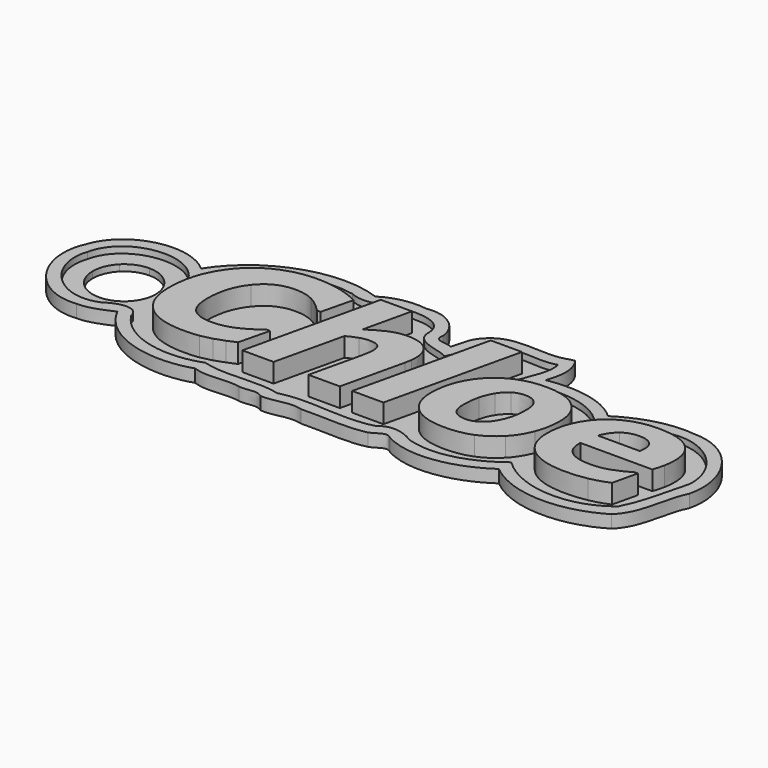
from build123d import *

# Parameters (mm, degrees)
F1_DEPTH = 4
F2_DEPTH = 1
F3_DEPTH = 2
F4_DEPTH = 1


# Not quite as in the source:
# - ends of sketch curves that miss each other by under 0.0002 mm in the source are joined


with BuildPart() as f1:
    # F0 (on Top) → F1 (new body)
    with BuildSketch(Plane.XY):
        with BuildLine():
            add(Edge.make_bspline(
                [(-23.2617298845, -10.9770997937), (-25.988726302, -10.9770997937), (-28.092665777, -10.3088950788), (-29.5735483095, -8.972486227)],
                knots=[0, 0, 0, 0, 1, 1, 1, 1], degree=3))
            add(Edge.make_bspline(
                [(-20.9049541001, -10.8281063081), (-21.4648019653, -10.9274351059), (-22.2503938934, -10.9770997937), (-23.2617298845, -10.9770997937)],
                knots=[0, 0, 0, 0, 1, 1, 1, 1], degree=3))
            add(Edge.make_bspline(
                [(-19.0764216423, -10.3946765976), (-19.7265679417, -10.5843038297), (-20.336078761, -10.7287803998), (-20.9049541001, -10.8281063081)],
                knots=[0, 0, 0, 0, 1, 1, 1, 1], degree=3))
            add(Edge.make_bspline(
                [(-17.5187839092, -9.8393456479), (-18.0605733589, -10.0650897109), (-18.579785744, -10.2502000274), (-19.0764216423, -10.3946765976)],
                knots=[0, 0, 0, 0, 1, 1, 1, 1], degree=3))
            add(Edge.make_bspline(
                [(-16.0965935386, -9.2433809518), (-16.5029338922, -9.4059159375), (-16.976997349, -9.6045706435), (-17.5187839092, -9.8393456479)],
                knots=[0, 0, 0, 0, 1, 1, 1, 1], degree=3))
            Line((-16.0965935386, -9.2433809518), (-14.9182056464, -4.4214742671))
            Line((-14.9182056464, -4.4214742671), (-15.4599950961, -4.4214742671))
            add(Edge.make_bspline(
                [(-18.561724439, -6.344820341), (-17.4691209551, -5.8391506117), (-16.4352113668, -5.1980352538), (-15.4599950961, -4.4214742671)],
                knots=[0, 0, 0, 0, 1, 1, 1, 1], degree=3))
            add(Edge.make_bspline(
                [(-22.0697958691, -7.0897785227), (-20.8236883411, -7.0897785227), (-19.6543308124, -6.8414591288), (-18.561724439, -6.344820341)],
                knots=[0, 0, 0, 0, 1, 1, 1, 1], degree=3))
            add(Edge.make_bspline(
                [(-25.2392512048, -6.0062042466), (-24.516868354, -6.7285870973), (-23.4603834348, -7.0897785227), (-22.0697958691, -7.0897785227)],
                knots=[0, 0, 0, 0, 1, 1, 1, 1], degree=3))
            add(Edge.make_bspline(
                [(-26.322825481, -2.5116743164), (-26.322825481, -4.1189778931), (-25.9616340556, -5.2838213958), (-25.2392512048, -6.0062042466)],
                knots=[0, 0, 0, 0, 1, 1, 1, 1], degree=3))
            add(Edge.make_bspline(
                [(-24.3723917839, 3.6646967461), (-25.6726809153, 2.0483651175), (-26.322825481, -0.0104248514), (-26.322825481, -2.5116743164)],
                knots=[0, 0, 0, 0, 1, 1, 1, 1], degree=3))
            add(Edge.make_bspline(
                [(-19.3879501135, 6.0891939001), (-21.4015946217, 6.0891939001), (-23.0630751785, 5.2810283747), (-24.3723917839, 3.6646967461)],
                knots=[0, 0, 0, 0, 1, 1, 1, 1], degree=3))
            add(Edge.make_bspline(
                [(-16.3945758866, 5.4390493344), (-17.2433768921, 5.8724790449), (-18.2411684937, 6.0891939001), (-19.3879501135, 6.0891939001)],
                knots=[0, 0, 0, 0, 1, 1, 1, 1], degree=3))
            add(Edge.make_bspline(
                [(-13.8346313703, 3.4073481445), (-14.6924633172, 4.3283857013), (-15.5457777707, 5.0056196239), (-16.3945758866, 5.4390493344)],
                knots=[0, 0, 0, 0, 1, 1, 1, 1], degree=3))
            Line((-13.8346313703, 3.4073481445), (-13.2386666742, 3.4073481445))
            Line((-13.2386666742, 3.4073481445), (-12.046737282, 8.2969761988))
            add(Edge.make_bspline(
                [(-15.2703678641, 9.5430900839), (-14.0784384719, 9.2631644176), (-13.0038951372, 8.8477931225), (-12.046737282, 8.2969761988)],
                knots=[0, 0, 0, 0, 1, 1, 1, 1], degree=3))
            add(Edge.make_bspline(
                [(-19.1441476351, 9.9765197943), (-17.7535600694, 9.9765197943), (-16.4623001458, 9.8320432242), (-15.2703678641, 9.5430900839)],
                knots=[0, 0, 0, 0, 1, 1, 1, 1], degree=3))
            add(Edge.make_bspline(
                [(-24.0879555591, 9.0148467574), (-22.5167717028, 9.6559621153), (-20.8688355355, 9.9765197943), (-19.1441476351, 9.9765197943)],
                knots=[0, 0, 0, 0, 1, 1, 1, 1], degree=3))
            add(Edge.make_bspline(
                [(-28.1107241925, 6.3465425017), (-26.9910313517, 7.4842966475), (-25.6501084739, 8.3737313994), (-24.0879555591, 9.0148467574)],
                knots=[0, 0, 0, 0, 1, 1, 1, 1], degree=3))
            add(Edge.make_bspline(
                [(-30.8196621945, 2.1747850059), (-30.1604855315, 3.7820856931), (-29.2575058123, 5.172671525), (-28.1107241925, 6.3465425017)],
                knots=[0, 0, 0, 0, 1, 1, 1, 1], degree=3))
            add(Edge.make_bspline(
                [(-31.7948767314, -3.2024526285), (-31.7948767314, -1.2249313082), (-31.4698050265, 0.5674814292), (-30.8196621945, 2.1747850059)],
                knots=[0, 0, 0, 0, 1, 1, 1, 1], degree=3))
            add(Edge.make_bspline(
                [(-29.5735483095, -8.972486227), (-31.0544337315, -7.6270493232), (-31.7948767314, -5.703704983), (-31.7948767314, -3.2024526285)],
                knots=[0, 0, 0, 0, 1, 1, 1, 1], degree=3))
        make_face()
    extrude(amount=F1_DEPTH)



with BuildPart() as f1b:
    # F0 (on Top) → F1, piece 2 (new body)
    with BuildSketch(Plane.XY):
        with BuildLine():
            add(Edge.make_bspline(
                [(3.4740269711, 1.1860197225), (3.4740269711, 0.969306601), (3.455966822, 0.6893838242), (3.4198471015, 0.346252548)],
                knots=[0, 0, 0, 0, 1, 1, 1, 1], degree=3))
            add(Edge.make_bspline(
                [(2.3498189486, 4.030405087), (3.0992911563, 3.3622003721), (3.4740269711, 2.4140723026), (3.4740269711, 1.1860197225)],
                knots=[0, 0, 0, 0, 1, 1, 1, 1], degree=3))
            add(Edge.make_bspline(
                [(-0.8467286336, 5.0462533703), (0.5348279907, 5.0462533703), (1.6003438514, 4.7076372759), (2.3498189486, 4.030405087)],
                knots=[0, 0, 0, 0, 1, 1, 1, 1], degree=3))
            add(Edge.make_bspline(
                [(-3.5827542588, 4.4909224207), (-2.7520116688, 4.8611430538), (-1.8400033197, 5.0462533703), (-0.8467286336, 5.0462533703)],
                knots=[0, 0, 0, 0, 1, 1, 1, 1], degree=3))
            add(Edge.make_bspline(
                [(-6.3187752608, 2.9468308108), (-5.3255005747, 3.6060045843), (-4.4134939593, 4.1207017875), (-3.5827542588, 4.4909224207)],
                knots=[0, 0, 0, 0, 1, 1, 1, 1], degree=3))
            Line((-6.3187752608, 2.9468308108), (-4.5850564189, 10.4912169976))
            Line((-4.5850564189, 10.4912169976), (-9.4882305964, 10.4912169976))
            Line((-9.4882305964, 10.4912169976), (-14.3507710276, -10.5843038297))
            Line((-14.3507710276, -10.5843038297), (-9.44759685, -10.5843038297))
            Line((-9.44759685, -10.5843038297), (-6.9553783265, 0.1972590624))
            add(Edge.make_bspline(
                [(-5.262293231, 0.9422172441), (-5.7679594928, 0.7796822585), (-6.332321384, 0.5313628646), (-6.9553783265, 0.1972590624)],
                knots=[0, 0, 0, 0, 1, 1, 1, 1], degree=3))
            add(Edge.make_bspline(
                [(-3.9213703532, 1.1995658457), (-4.3096494018, 1.1995658457), (-4.7566235018, 1.1137831712), (-5.262293231, 0.9422172441)],
                knots=[0, 0, 0, 0, 1, 1, 1, 1], degree=3))
            add(Edge.make_bspline(
                [(-2.2824651274, 0.7932237585), (-2.5804457417, 1.0641184833), (-3.1267474836, 1.1995658457), (-3.9213703532, 1.1995658457)],
                knots=[0, 0, 0, 0, 1, 1, 1, 1], degree=3))
            add(Edge.make_bspline(
                [(-1.8219431705, -0.5070653729), (-1.8219431705, 0.0979302646), (-1.9754506821, 0.5313599751), (-2.2824651274, 0.7932237585)],
                knots=[0, 0, 0, 0, 1, 1, 1, 1], degree=3))
            add(Edge.make_bspline(
                [(-1.9303029097, -1.5770935259), (-1.8580628909, -1.1797835359), (-1.8219431705, -0.8231078701), (-1.8219431705, -0.5070653729)],
                knots=[0, 0, 0, 0, 1, 1, 1, 1], degree=3))
            add(Edge.make_bspline(
                [(-2.2282852578, -3.0399176429), (-2.1018671031, -2.4620113623), (-2.0025394611, -1.9744035159), (-1.9303029097, -1.5770935259)],
                knots=[0, 0, 0, 0, 1, 1, 1, 1], degree=3))
            Line((-2.2282852578, -3.0399176429), (-3.9755502228, -10.5843038297))
            Line((-3.9755502228, -10.5843038297), (0.9547162012, -10.5843038297))
            Line((0.9547162012, -10.5843038297), (3.2437659927, -0.6831464818))
            add(Edge.make_bspline(
                [(3.4198471015, 0.346252548), (3.3837273811, 0.0031212718), (3.3250334855, -0.3400117381), (3.2437659927, -0.6831464818)],
                knots=[0, 0, 0, 0, 1, 1, 1, 1], degree=3))
        make_face()
    extrude(amount=F1_DEPTH)


with BuildPart() as f1c:
    # F0 (on Top) → F1, piece 3 (new body)
    with BuildSketch(Plane.XY):
        Polygon((7.7947502131, -10.5843038297), (12.6708367675, 10.4912169976), (7.7676625899, 10.4912169976), (2.8915760355, -10.5843038297), align=None)
    extrude(amount=F1_DEPTH)


with BuildPart() as f1d:
    # F0 (on Top) → F1, piece 4 (new body)
    with BuildSketch(Plane.XY):
        with BuildLine():
            add(Edge.make_bspline(
                [(27.7802611998, -0.9404950834), (27.7802611998, -2.36719948), (27.5409710136, -3.7036065981), (27.0623906413, -4.9497175936)],
                knots=[0, 0, 0, 0, 1, 1, 1, 1], degree=3))
            add(Edge.make_bspline(
                [(25.9652702419, 3.4886156373), (27.1752644065, 2.4231015103), (27.7802611998, 0.9467312701), (27.7802611998, -0.9404950834)],
                knots=[0, 0, 0, 0, 1, 1, 1, 1], degree=3))
            add(Edge.make_bspline(
                [(20.7505722163, 5.1004332399), (23.0260776184, 5.1004332399), (24.7643099083, 4.5631607057), (25.9652702419, 3.4886156373)],
                knots=[0, 0, 0, 0, 1, 1, 1, 1], degree=3))
            add(Edge.make_bspline(
                [(16.5381763509, 4.3012951886), (17.7933177099, 4.8340536969), (19.1974496651, 5.1004332399), (20.7505722163, 5.1004332399)],
                knots=[0, 0, 0, 0, 1, 1, 1, 1], degree=3))
            add(Edge.make_bspline(
                [(13.3822671384, 2.1476927595), (14.2400956179, 3.0597028423), (15.2920653554, 3.7775705113), (16.5381763509, 4.3012951886)],
                knots=[0, 0, 0, 0, 1, 1, 1, 1], degree=3))
            add(Edge.make_bspline(
                [(11.3776535717, -1.0759378226), (11.8291416976, 0.1430809265), (12.4973464125, 1.2176242612), (13.3822671384, 2.1476927595)],
                knots=[0, 0, 0, 0, 1, 1, 1, 1], degree=3))
            add(Edge.make_bspline(
                [(10.7004213828, -4.9361714704), (10.7004213828, -3.5817042031), (10.9261654458, -2.2949594612), (11.3776535717, -1.0759378226)],
                knots=[0, 0, 0, 0, 1, 1, 1, 1], degree=3))
            add(Edge.make_bspline(
                [(12.5154077175, -9.4330081839), (11.3054170203, -8.349432174), (10.7004213828, -6.8504866028), (10.7004213828, -4.9361714704)],
                knots=[0, 0, 0, 0, 1, 1, 1, 1], degree=3))
            add(Edge.make_bspline(
                [(17.730105743, -11.0583672865), (15.4636312824, -11.0583672865), (13.7253984146, -10.5165807263), (12.5154077175, -9.4330081839)],
                knots=[0, 0, 0, 0, 1, 1, 1, 1], degree=3))
            add(Edge.make_bspline(
                [(21.9018678621, -10.3134091048), (20.7099355804, -10.8100478926), (19.3193480148, -11.0583672865), (17.730105743, -11.0583672865)],
                knots=[0, 0, 0, 0, 1, 1, 1, 1], degree=3))
            add(Edge.make_bspline(
                [(25.0442355746, -8.1598066757), (24.1412564332, -9.089875174), (23.0938001438, -9.807742843), (21.9018678621, -10.3134091048)],
                knots=[0, 0, 0, 0, 1, 1, 1, 1], degree=3))
            add(Edge.make_bspline(
                [(27.0623906413, -4.9497175936), (26.5838131585, -6.1958285891), (25.9110949955, -7.2658578978), (25.0442355746, -8.1598066757)],
                knots=[0, 0, 0, 0, 1, 1, 1, 1], degree=3))
        make_face()
        with BuildLine():
            add(Edge.make_bspline(
                [(21.4413505284, -5.9249367538), (21.8567189339, -5.2928488698), (22.1682456715, -4.6020694019), (22.375931319, -3.8525971942)],
                knots=[0, 0, 0, 0, 1, 1, 1, 1], degree=3))
            add(Edge.make_bspline(
                [(20.0597939042, -7.2658596316), (20.6015804644, -6.9407867708), (21.0620989539, -6.4938120929), (21.4413505284, -5.9249367538)],
                knots=[0, 0, 0, 0, 1, 1, 1, 1], degree=3))
            add(Edge.make_bspline(
                [(18.3667088088, -7.7399230884), (18.9536425634, -7.7399230884), (19.5180044545, -7.5819021288), (20.0597939042, -7.2658596316)],
                knots=[0, 0, 0, 0, 1, 1, 1, 1], degree=3))
            add(Edge.make_bspline(
                [(16.4704549813, -7.0762323995), (16.9309740487, -7.5186930514), (17.5630584652, -7.7399230884), (18.3667088088, -7.7399230884)],
                knots=[0, 0, 0, 0, 1, 1, 1, 1], degree=3))
            add(Edge.make_bspline(
                [(15.7796720459, -4.8413624776), (15.7796720459, -5.8797878256), (16.0099330244, -6.6247442736), (16.4704549813, -7.0762323995)],
                knots=[0, 0, 0, 0, 1, 1, 1, 1], degree=3))
            add(Edge.make_bspline(
                [(16.0912005172, -2.2543257148), (15.8835148697, -3.0940957788), (15.7796720459, -3.9564417517), (15.7796720459, -4.8413624776)],
                knots=[0, 0, 0, 0, 1, 1, 1, 1], degree=3))
            add(Edge.make_bspline(
                [(16.9716060613, -0.1413570321), (16.6013854282, -0.7102323712), (16.3079171062, -1.4145556507), (16.0912005172, -2.2543257148)],
                knots=[0, 0, 0, 0, 1, 1, 1, 1], degree=3))
            add(Edge.make_bspline(
                [(18.3396165623, 1.2808333386), (17.8249193591, 0.9467324259), (17.3689160514, 0.472668969), (16.9716060613, -0.1413570321)],
                knots=[0, 0, 0, 0, 1, 1, 1, 1], degree=3))
            add(Edge.make_bspline(
                [(20.1546075203, 1.7819890419), (19.4683415004, 1.7819890419), (18.8633447071, 1.6149371408), (18.3396165623, 1.2808333386)],
                knots=[0, 0, 0, 0, 1, 1, 1, 1], degree=3))
            add(Edge.make_bspline(
                [(22.0914950941, 1.0234847369), (21.6851547406, 1.5291544662), (21.0395253566, 1.7819890419), (20.1546075203, 1.7819890419)],
                knots=[0, 0, 0, 0, 1, 1, 1, 1], degree=3))
            add(Edge.make_bspline(
                [(22.7010059134, -1.1165761922), (22.7010059134, -0.1865076939), (22.4978354477, 0.5268459491), (22.0914950941, 1.0234847369)],
                knots=[0, 0, 0, 0, 1, 1, 1, 1], degree=3))
            add(Edge.make_bspline(
                [(22.375931319, -3.8525971942), (22.5926479079, -3.1031249865), (22.7010059134, -2.1911183711), (22.7010059134, -1.1165761922)],
                knots=[0, 0, 0, 0, 1, 1, 1, 1], degree=3))
        make_face(mode=Mode.SUBTRACT)
    extrude(amount=F1_DEPTH)


with BuildPart() as f1e:
    # F0 (on Top) → F1, piece 5 (new body)
    with BuildSketch(Plane.XY):
        with BuildLine():
            add(Edge.make_bspline(
                [(36.644169239, -10.9906459169), (34.0526184502, -10.9906459169), (32.0525206432, -10.4172536623), (30.6438746621, -9.270468575)],
                knots=[0, 0, 0, 0, 1, 1, 1, 1], degree=3))
            add(Edge.make_bspline(
                [(39.9897056835, -10.6655713225), (38.942249972, -10.8822879114), (37.8270711572, -10.9906459169), (36.644169239, -10.9906459169)],
                knots=[0, 0, 0, 0, 1, 1, 1, 1], degree=3))
            add(Edge.make_bspline(
                [(42.9830799104, -9.7309905319), (42.0349501071, -10.1463589374), (41.0371585055, -10.457885675), (39.9897056835, -10.6655713225)],
                knots=[0, 0, 0, 0, 1, 1, 1, 1], degree=3))
            Line((42.9830799104, -9.7309905319), (43.8905730777, -5.8165770145))
            Line((43.8905730777, -5.8165770145), (43.348783628, -5.8165770145))
            add(Edge.make_bspline(
                [(40.8565651045, -7.0220525299), (41.8137194922, -6.6608628382), (42.6444591927, -6.2590376664), (43.348783628, -5.8165770145)],
                knots=[0, 0, 0, 0, 1, 1, 1, 1], degree=3))
            add(Edge.make_bspline(
                [(37.8360986312, -7.5638419796), (38.9016127582, -7.5638419796), (39.9084353012, -7.383245689), (40.8565651045, -7.0220525299)],
                knots=[0, 0, 0, 0, 1, 1, 1, 1], degree=3))
            add(Edge.make_bspline(
                [(34.4363869403, -6.6698903122), (35.1768282065, -7.2658578978), (36.3100654368, -7.5638419796), (37.8360986312, -7.5638419796)],
                knots=[0, 0, 0, 0, 1, 1, 1, 1], degree=3))
            add(Edge.make_bspline(
                [(33.3257204177, -4.1912179119), (33.3257204177, -5.2477016753), (33.6959427845, -6.0739256162), (34.4363869403, -6.6698903122)],
                knots=[0, 0, 0, 0, 1, 1, 1, 1], degree=3))
            add(Edge.make_bspline(
                [(33.3257204177, -4.0422244263), (33.3257204177, -4.0873721986), (33.3257204177, -4.1370363086), (33.3257204177, -4.1912179119)],
                knots=[0, 0, 0, 0, 1, 1, 1, 1], degree=3))
            add(Edge.make_bspline(
                [(33.3257204177, -3.8796894406), (33.3257204177, -3.9338675765), (33.3257204177, -3.9880462903), (33.3257204177, -4.0422244263)],
                knots=[0, 0, 0, 0, 1, 1, 1, 1], degree=3))
            Line((33.3257204177, -3.8796894406), (44.6219851362, -3.8796894406))
            add(Edge.make_bspline(
                [(45.0960485931, -2.1324244756), (44.9786613798, -2.7193616976), (44.8206398423, -3.30178316), (44.6219851362, -3.8796894406)],
                knots=[0, 0, 0, 0, 1, 1, 1, 1], degree=3))
            add(Edge.make_bspline(
                [(45.2856712019, -0.3309842641), (45.2856712019, -0.9450073756), (45.2224638583, -1.5454872535), (45.0960485931, -2.1324244756)],
                knots=[0, 0, 0, 0, 1, 1, 1, 1], degree=3))
            add(Edge.make_bspline(
                [(43.55195236, 3.7188766157), (44.7077649213, 2.8068665329), (45.2856712019, 1.4569127137), (45.2856712019, -0.3309842641)],
                knots=[0, 0, 0, 0, 1, 1, 1, 1], degree=3))
            add(Edge.make_bspline(
                [(38.4320679505, 5.1004332399), (40.6985424111, 5.1004332399), (42.4051707402, 4.6399141726), (43.55195236, 3.7188766157)],
                knots=[0, 0, 0, 0, 1, 1, 1, 1], degree=3))
            add(Edge.make_bspline(
                [(34.328027201, 4.3554750582), (35.5741381965, 4.852113846), (36.942151587, 5.1004332399), (38.4320679505, 5.1004332399)],
                knots=[0, 0, 0, 0, 1, 1, 1, 1], degree=3))
            add(Edge.make_bspline(
                [(31.212751735, 2.3373199915), (32.0434914354, 3.1861181075), (33.0819162055, 3.8588362704), (34.328027201, 4.3554750582)],
                knots=[0, 0, 0, 0, 1, 1, 1, 1], degree=3))
            add(Edge.make_bspline(
                [(29.2216842915, -0.7102341049), (29.6822033588, 0.4455784563), (30.345892314, 1.4614296292), (31.212751735, 2.3373199915)],
                knots=[0, 0, 0, 0, 1, 1, 1, 1], degree=3))
            add(Edge.make_bspline(
                [(28.5309059794, -4.5162878831), (28.5309059794, -3.1347312589), (28.7611652241, -1.8660466662), (29.2216842915, -0.7102341049)],
                knots=[0, 0, 0, 0, 1, 1, 1, 1], degree=3))
            add(Edge.make_bspline(
                [(30.6438746621, -9.270468575), (29.235228681, -8.1236869552), (28.5309059794, -6.5389598653), (28.5309059794, -4.5162878831)],
                knots=[0, 0, 0, 0, 1, 1, 1, 1], degree=3))
        make_face()
        with BuildLine():
            add(Edge.make_bspline(
                [(40.3689555244, -1.0217625762), (40.3960477708, -0.8592247011), (40.41410792, -0.7102323712), (40.423135394, -0.5747867425)],
                knots=[0, 0, 0, 0, 1, 1, 1, 1], degree=3))
            Line((40.3689555244, -1.0217625762), (33.7997884978, -1.0217625762))
            add(Edge.make_bspline(
                [(35.3438847309, 1.2401995922), (34.6666496524, 0.698413032), (34.1519507154, -0.0555743575), (33.7997884978, -1.0217625762)],
                knots=[0, 0, 0, 0, 1, 1, 1, 1], degree=3))
            add(Edge.make_bspline(
                [(37.8767370008, 2.0528791435), (36.8744319512, 2.0528791435), (36.0301478612, 1.7819861523), (35.3438847309, 1.2401995922)],
                knots=[0, 0, 0, 0, 1, 1, 1, 1], degree=3))
            add(Edge.make_bspline(
                [(39.7865369515, 1.4840020706), (39.344079767, 1.8632536451), (38.7074795908, 2.0528791435), (37.8767370008, 2.0528791435)],
                knots=[0, 0, 0, 0, 1, 1, 1, 1], degree=3))
            add(Edge.make_bspline(
                [(40.4502276404, -0.1549031553), (40.4502276404, 0.5584522215), (40.2289976034, 1.1047539634), (39.7865369515, 1.4840020706)],
                knots=[0, 0, 0, 0, 1, 1, 1, 1], degree=3))
            add(Edge.make_bspline(
                [(40.423135394, -0.5747867425), (40.441196699, -0.4393411138), (40.4502276404, -0.2993797254), (40.4502276404, -0.1549031553)],
                knots=[0, 0, 0, 0, 1, 1, 1, 1], degree=3))
        make_face(mode=Mode.SUBTRACT)
    extrude(amount=F1_DEPTH)


with BuildPart() as f1_1:
    add(f1.part)

    add(f1b.part)  # F2 merges F1b

    add(f1c.part)  # F2 merges F1c

    add(f1d.part)  # F2 merges F1d

    add(f1e.part)  # F2 merges F1e
    # F0 (on Top) → F2 (join)
    with BuildSketch(Plane.XY):
        with BuildLine():
            Line((15.8580130213, 13.5759327795), (15.6241412845, 13.5154329268))
            add(Edge.make_bspline(
                [(15.6241412845, 13.5154329268), (12.2612861445, 12.5592014554), (7.5632918128, 14.7974694663), (5.2137005593, 11.4512210412)],
                knots=[0, 0, 0, 0, 1, 1, 1, 1], degree=3))
            add(Edge.make_bspline(
                [(5.2137005593, 11.4512210412), (4.5835376812, 9.8969166716), (4.4090839564, 8.1808077899), (3.555830761, 6.7078772479)],
                knots=[0, 0, 0, 0, 1, 1, 1, 1], degree=3))
            add(Edge.make_bspline(
                [(3.555830761, 6.7078772479), (1.7174230406, 7.7203274423), (-2.0104377062, 7.48397302), (-1.8503021875, 10.4823264874)],
                knots=[0, 0, 0, 0, 1, 1, 1, 1], degree=3))
            add(Edge.make_bspline(
                [(-1.8503021875, 10.4823264874), (-2.0797494739, 13.9126625879), (-6.4930255625, 13.6147449654), (-8.9359741082, 13.3420610427)],
                knots=[0, 0, 0, 0, 1, 1, 1, 1], degree=3))
            add(Edge.make_bspline(
                [(-8.9359741082, 13.3420610427), (-11.0645462605, 12.5389747356), (-13.3300822013, 11.5014064226), (-15.5719655938, 12.5591783392)],
                knots=[0, 0, 0, 0, 1, 1, 1, 1], degree=3))
            add(Edge.make_bspline(
                [(-15.5719655938, 12.5591783392), (-22.8393821049, 13.9938191227), (-30.6726751995, 9.9797052137), (-33.8645024431, 3.2494687719)],
                knots=[0, 0, 0, 0, 1, 1, 1, 1], degree=3))
            add(Edge.make_bspline(
                [(-33.8645024431, 3.2494687719), (-37.1800894725, 8.5080645585), (-46.5444273647, 7.1839980511), (-47.8787297482, 1.0082742436)],
                knots=[0, 0, 0, 0, 1, 1, 1, 1], degree=3))
            add(Edge.make_bspline(
                [(-47.8787297482, 1.0082742436), (-49.7924455918, -4.4794405787), (-43.6641378389, -10.7966265972), (-38.1419150767, -8.4106919735)],
                knots=[0, 0, 0, 0, 1, 1, 1, 1], degree=3))
            add(Edge.make_bspline(
                [(-38.1419150767, -8.4106919735), (-36.6391599474, -7.3409180993), (-33.7268405438, -6.3989077456), (-33.107805829, -8.9362260753)],
                knots=[0, 0, 0, 0, 1, 1, 1, 1], degree=3))
            add(Edge.make_bspline(
                [(-33.107805829, -8.9362260753), (-30.063825505, -13.7507031969), (-23.309238404, -14.8906210238), (-18.235752934, -12.9806685059)],
                knots=[0, 0, 0, 0, 1, 1, 1, 1], degree=3))
            add(Edge.make_bspline(
                [(-18.235752934, -12.9806685059), (-14.3543216838, -14.1260094053), (-10.2215659271, -12.7657382252), (-6.3046928405, -13.7698711924)],
                knots=[0, 0, 0, 0, 1, 1, 1, 1], degree=3))
            add(Edge.make_bspline(
                [(-6.3046928405, -13.7698711924), (-1.4698456783, -12.5003960239), (3.7343529459, -14.3804083733), (8.5601385376, -13.0222037861)],
                knots=[0, 0, 0, 0, 1, 1, 1, 1], degree=3))
            add(Edge.make_bspline(
                [(8.5601385376, -13.0222037861), (10.2158446549, -11.6093570042), (12.4228317546, -12.2589791426), (14.0204513557, -13.3147723081)],
                knots=[0, 0, 0, 0, 1, 1, 1, 1], degree=3))
            add(Edge.make_bspline(
                [(14.0204513557, -13.3147723081), (18.6889863368, -14.851808838), (23.8157316498, -13.1253253828), (27.5434583223, -10.176015354)],
                knots=[0, 0, 0, 0, 1, 1, 1, 1], degree=3))
            add(Edge.make_bspline(
                [(27.5434583223, -10.176015354), (32.0649369596, -14.6914144173), (40.2710258377, -15.2455664381), (45.1091000285, -11.0826069876)],
                knots=[0, 0, 0, 0, 1, 1, 1, 1], degree=3))
            add(Edge.make_bspline(
                [(45.1091000285, -11.0826069876), (46.7440801149, -7.9685659293), (47.2377831388, -4.3614737254), (48.2054109221, -1.0342638449)],
                knots=[0, 0, 0, 0, 1, 1, 1, 1], degree=3))
            add(Edge.make_bspline(
                [(48.2054109221, -1.0342638449), (48.4801383214, 4.1566799209), (43.480028456, 8.8316504664), (38.2879982264, 7.9296081111)],
                knots=[0, 0, 0, 0, 1, 1, 1, 1], degree=3))
            add(Edge.make_bspline(
                [(38.2879982264, 7.9296081111), (34.8822624404, 7.8320297914), (31.6595796246, 6.3816052316), (28.9096611324, 4.4450135457)],
                knots=[0, 0, 0, 0, 1, 1, 1, 1], degree=3))
            add(Edge.make_bspline(
                [(28.9096611324, 4.4450135457), (25.3301188767, 8.682365716), (19.1984731371, 8.343555445), (14.3446197932, 7.0103718882)],
                knots=[0, 0, 0, 0, 1, 1, 1, 1], degree=3))
            add(Edge.make_bspline(
                [(14.3446197932, 7.0103718882), (14.9786708247, 9.126706297), (16.3623171581, 11.287604215), (15.8580130213, 13.5759327795)],
                knots=[0, 0, 0, 0, 1, 1, 1, 1], degree=3))
        make_face()
        with BuildLine():
            add(Edge.make_bspline(
                [(-36.9707781747, 2.3684292645), (-36.0457646226, 1.4434151346), (-35.5260980032, 0.1888262539), (-35.5260985811, -1.1193408959)],
                knots=[0, 0, 0, 0, 1, 1, 1, 1], degree=3))
            add(Edge.make_bspline(
                [(-35.5260985811, -1.1193408959), (-35.5260997369, -3.8434564506), (-37.7344316246, -6.0517883382), (-40.4585471792, -6.051789494)],
                knots=[0, 0, 0, 0, 1, 1, 1, 1], degree=3))
            add(Edge.make_bspline(
                [(-40.4585471792, -6.051789494), (-43.1826627339, -6.0517883382), (-45.3909946215, -3.8434564506), (-45.3909957774, -1.1193408959)],
                knots=[0, 0, 0, 0, 1, 1, 1, 1], degree=3))
            add(Edge.make_bspline(
                [(-45.3909957774, -1.1193408959), (-45.3909963553, 0.1888262539), (-44.8713297359, 1.4434151346), (-43.9463161838, 2.3684292645)],
                knots=[0, 0, 0, 0, 1, 1, 1, 1], degree=3))
            add(Edge.make_bspline(
                [(-43.9463161838, 2.3684292645), (-43.0213026318, 3.2934439724), (-41.7667143291, 3.8131117476), (-40.4585471792, 3.8131123255)],
                knots=[0, 0, 0, 0, 1, 1, 1, 1], degree=3))
            add(Edge.make_bspline(
                [(-40.4585471792, 3.8131123255), (-39.1503800294, 3.8131117476), (-37.8957917267, 3.2934439724), (-36.9707781747, 2.3684292645)],
                knots=[0, 0, 0, 0, 1, 1, 1, 1], degree=3))
        make_face(mode=Mode.SUBTRACT)
        with BuildLine():
            add(Edge.make_bspline(
                [(-20.9049541001, -10.8281063081), (-21.4648019653, -10.9274351059), (-22.2503938934, -10.9770997937), (-23.2617298845, -10.9770997937)],
                knots=[0, 0, 0, 0, 1, 1, 1, 1], degree=3))
            add(Edge.make_bspline(
                [(-23.2617298845, -10.9770997937), (-25.988726302, -10.9770997937), (-28.092665777, -10.3088950788), (-29.5735483095, -8.972486227)],
                knots=[0, 0, 0, 0, 1, 1, 1, 1], degree=3))
            add(Edge.make_bspline(
                [(-29.5735483095, -8.972486227), (-31.0544337315, -7.6270493232), (-31.7948767314, -5.703704983), (-31.7948767314, -3.2024526285)],
                knots=[0, 0, 0, 0, 1, 1, 1, 1], degree=3))
            add(Edge.make_bspline(
                [(-31.7948767314, -3.2024526285), (-31.7948767314, -1.2249313082), (-31.4698050265, 0.5674814292), (-30.8196621945, 2.1747850059)],
                knots=[0, 0, 0, 0, 1, 1, 1, 1], degree=3))
            add(Edge.make_bspline(
                [(-30.8196621945, 2.1747850059), (-30.1604855315, 3.7820856931), (-29.2575058123, 5.172671525), (-28.1107241925, 6.3465425017)],
                knots=[0, 0, 0, 0, 1, 1, 1, 1], degree=3))
            add(Edge.make_bspline(
                [(-28.1107241925, 6.3465425017), (-26.9910313517, 7.4842966475), (-25.6501084739, 8.3737313994), (-24.0879555591, 9.0148467574)],
                knots=[0, 0, 0, 0, 1, 1, 1, 1], degree=3))
            add(Edge.make_bspline(
                [(-24.0879555591, 9.0148467574), (-22.5167717028, 9.6559621153), (-20.8688355355, 9.9765197943), (-19.1441476351, 9.9765197943)],
                knots=[0, 0, 0, 0, 1, 1, 1, 1], degree=3))
            add(Edge.make_bspline(
                [(-19.1441476351, 9.9765197943), (-17.7535600694, 9.9765197943), (-16.4623001458, 9.8320432242), (-15.2703678641, 9.5430900839)],
                knots=[0, 0, 0, 0, 1, 1, 1, 1], degree=3))
            add(Edge.make_bspline(
                [(-15.2703678641, 9.5430900839), (-14.0784384719, 9.2631644176), (-13.0038951372, 8.8477931225), (-12.046737282, 8.2969761988)],
                knots=[0, 0, 0, 0, 1, 1, 1, 1], degree=3))
            Line((-12.046737282, 8.2969761988), (-13.2386666742, 3.4073481445))
            Line((-13.2386666742, 3.4073481445), (-13.8346313703, 3.4073481445))
            add(Edge.make_bspline(
                [(-13.8346313703, 3.4073481445), (-14.6924633172, 4.3283857013), (-15.5457777707, 5.0056196239), (-16.3945758866, 5.4390493344)],
                knots=[0, 0, 0, 0, 1, 1, 1, 1], degree=3))
            add(Edge.make_bspline(
                [(-16.3945758866, 5.4390493344), (-17.2433768921, 5.8724790449), (-18.2411684937, 6.0891939001), (-19.3879501135, 6.0891939001)],
                knots=[0, 0, 0, 0, 1, 1, 1, 1], degree=3))
            add(Edge.make_bspline(
                [(-19.3879501135, 6.0891939001), (-21.4015946217, 6.0891939001), (-23.0630751785, 5.2810283747), (-24.3723917839, 3.6646967461)],
                knots=[0, 0, 0, 0, 1, 1, 1, 1], degree=3))
            add(Edge.make_bspline(
                [(-24.3723917839, 3.6646967461), (-25.6726809153, 2.0483651175), (-26.322825481, -0.0104248514), (-26.322825481, -2.5116743164)],
                knots=[0, 0, 0, 0, 1, 1, 1, 1], degree=3))
            add(Edge.make_bspline(
                [(-26.322825481, -2.5116743164), (-26.322825481, -4.1189778931), (-25.9616340556, -5.2838213958), (-25.2392512048, -6.0062042466)],
                knots=[0, 0, 0, 0, 1, 1, 1, 1], degree=3))
            add(Edge.make_bspline(
                [(-25.2392512048, -6.0062042466), (-24.516868354, -6.7285870973), (-23.4603834348, -7.0897785227), (-22.0697958691, -7.0897785227)],
                knots=[0, 0, 0, 0, 1, 1, 1, 1], degree=3))
            add(Edge.make_bspline(
                [(-22.0697958691, -7.0897785227), (-20.8236883411, -7.0897785227), (-19.6543308124, -6.8414591288), (-18.561724439, -6.344820341)],
                knots=[0, 0, 0, 0, 1, 1, 1, 1], degree=3))
            add(Edge.make_bspline(
                [(-18.561724439, -6.344820341), (-17.4691209551, -5.8391506117), (-16.4352113668, -5.1980352538), (-15.4599950961, -4.4214742671)],
                knots=[0, 0, 0, 0, 1, 1, 1, 1], degree=3))
            Line((-15.4599950961, -4.4214742671), (-14.9182056464, -4.4214742671))
            Line((-14.9182056464, -4.4214742671), (-16.0965935386, -9.2433809518))
            add(Edge.make_bspline(
                [(-16.0965935386, -9.2433809518), (-16.5029338922, -9.4059159375), (-16.976997349, -9.6045706435), (-17.5187839092, -9.8393456479)],
                knots=[0, 0, 0, 0, 1, 1, 1, 1], degree=3))
            add(Edge.make_bspline(
                [(-17.5187839092, -9.8393456479), (-18.0605733589, -10.0650897109), (-18.579785744, -10.2502000274), (-19.0764216423, -10.3946765976)],
                knots=[0, 0, 0, 0, 1, 1, 1, 1], degree=3))
            add(Edge.make_bspline(
                [(-19.0764216423, -10.3946765976), (-19.7265679417, -10.5843038297), (-20.336078761, -10.7287803998), (-20.9049541001, -10.8281063081)],
                knots=[0, 0, 0, 0, 1, 1, 1, 1], degree=3))
        make_face(mode=Mode.SUBTRACT)
        with BuildLine():
            add(Edge.make_bspline(
                [(25.9652702419, 3.4886156373), (27.1752644065, 2.4231015103), (27.7802611998, 0.9467312701), (27.7802611998, -0.9404950834)],
                knots=[0, 0, 0, 0, 1, 1, 1, 1], degree=3))
            add(Edge.make_bspline(
                [(27.7802611998, -0.9404950834), (27.7802611998, -2.36719948), (27.5409710136, -3.7036065981), (27.0623906413, -4.9497175936)],
                knots=[0, 0, 0, 0, 1, 1, 1, 1], degree=3))
            add(Edge.make_bspline(
                [(27.0623906413, -4.9497175936), (26.5838131585, -6.1958285891), (25.9110949955, -7.2658578978), (25.0442355746, -8.1598066757)],
                knots=[0, 0, 0, 0, 1, 1, 1, 1], degree=3))
            add(Edge.make_bspline(
                [(25.0442355746, -8.1598066757), (24.1412564332, -9.089875174), (23.0938001438, -9.807742843), (21.9018678621, -10.3134091048)],
                knots=[0, 0, 0, 0, 1, 1, 1, 1], degree=3))
            add(Edge.make_bspline(
                [(21.9018678621, -10.3134091048), (20.7099355804, -10.8100478926), (19.3193480148, -11.0583672865), (17.730105743, -11.0583672865)],
                knots=[0, 0, 0, 0, 1, 1, 1, 1], degree=3))
            add(Edge.make_bspline(
                [(17.730105743, -11.0583672865), (15.4636312824, -11.0583672865), (13.7253984146, -10.5165807263), (12.5154077175, -9.4330081839)],
                knots=[0, 0, 0, 0, 1, 1, 1, 1], degree=3))
            add(Edge.make_bspline(
                [(12.5154077175, -9.4330081839), (11.3054170203, -8.349432174), (10.7004213828, -6.8504866028), (10.7004213828, -4.9361714704)],
                knots=[0, 0, 0, 0, 1, 1, 1, 1], degree=3))
            add(Edge.make_bspline(
                [(10.7004213828, -4.9361714704), (10.7004213828, -3.5817042031), (10.9261654458, -2.2949594612), (11.3776535717, -1.0759378226)],
                knots=[0, 0, 0, 0, 1, 1, 1, 1], degree=3))
            add(Edge.make_bspline(
                [(11.3776535717, -1.0759378226), (11.8291416976, 0.1430809265), (12.4973464125, 1.2176242612), (13.3822671384, 2.1476927595)],
                knots=[0, 0, 0, 0, 1, 1, 1, 1], degree=3))
            add(Edge.make_bspline(
                [(13.3822671384, 2.1476927595), (14.2400956179, 3.0597028423), (15.2920653554, 3.7775705113), (16.5381763509, 4.3012951886)],
                knots=[0, 0, 0, 0, 1, 1, 1, 1], degree=3))
            add(Edge.make_bspline(
                [(16.5381763509, 4.3012951886), (17.7933177099, 4.8340536969), (19.1974496651, 5.1004332399), (20.7505722163, 5.1004332399)],
                knots=[0, 0, 0, 0, 1, 1, 1, 1], degree=3))
            add(Edge.make_bspline(
                [(20.7505722163, 5.1004332399), (23.0260776184, 5.1004332399), (24.7643099083, 4.5631607057), (25.9652702419, 3.4886156373)],
                knots=[0, 0, 0, 0, 1, 1, 1, 1], degree=3))
        make_face(mode=Mode.SUBTRACT)
        with BuildLine():
            add(Edge.make_bspline(
                [(39.9897056835, -10.6655713225), (38.942249972, -10.8822879114), (37.8270711572, -10.9906459169), (36.644169239, -10.9906459169)],
                knots=[0, 0, 0, 0, 1, 1, 1, 1], degree=3))
            add(Edge.make_bspline(
                [(36.644169239, -10.9906459169), (34.0526184502, -10.9906459169), (32.0525206432, -10.4172536623), (30.6438746621, -9.270468575)],
                knots=[0, 0, 0, 0, 1, 1, 1, 1], degree=3))
            add(Edge.make_bspline(
                [(30.6438746621, -9.270468575), (29.235228681, -8.1236869552), (28.5309059794, -6.5389598653), (28.5309059794, -4.5162878831)],
                knots=[0, 0, 0, 0, 1, 1, 1, 1], degree=3))
            add(Edge.make_bspline(
                [(28.5309059794, -4.5162878831), (28.5309059794, -3.1347312589), (28.7611652241, -1.8660466662), (29.2216842915, -0.7102341049)],
                knots=[0, 0, 0, 0, 1, 1, 1, 1], degree=3))
            add(Edge.make_bspline(
                [(29.2216842915, -0.7102341049), (29.6822033588, 0.4455784563), (30.345892314, 1.4614296292), (31.212751735, 2.3373199915)],
                knots=[0, 0, 0, 0, 1, 1, 1, 1], degree=3))
            add(Edge.make_bspline(
                [(31.212751735, 2.3373199915), (32.0434914354, 3.1861181075), (33.0819162055, 3.8588362704), (34.328027201, 4.3554750582)],
                knots=[0, 0, 0, 0, 1, 1, 1, 1], degree=3))
            add(Edge.make_bspline(
                [(34.328027201, 4.3554750582), (35.5741381965, 4.852113846), (36.942151587, 5.1004332399), (38.4320679505, 5.1004332399)],
                knots=[0, 0, 0, 0, 1, 1, 1, 1], degree=3))
            add(Edge.make_bspline(
                [(38.4320679505, 5.1004332399), (40.6985424111, 5.1004332399), (42.4051707402, 4.6399141726), (43.55195236, 3.7188766157)],
                knots=[0, 0, 0, 0, 1, 1, 1, 1], degree=3))
            add(Edge.make_bspline(
                [(43.55195236, 3.7188766157), (44.7077649213, 2.8068665329), (45.2856712019, 1.4569127137), (45.2856712019, -0.3309842641)],
                knots=[0, 0, 0, 0, 1, 1, 1, 1], degree=3))
            add(Edge.make_bspline(
                [(45.2856712019, -0.3309842641), (45.2856712019, -0.9450073756), (45.2224638583, -1.5454872535), (45.0960485931, -2.1324244756)],
                knots=[0, 0, 0, 0, 1, 1, 1, 1], degree=3))
            add(Edge.make_bspline(
                [(45.0960485931, -2.1324244756), (44.9786613798, -2.7193616976), (44.8206398423, -3.30178316), (44.6219851362, -3.8796894406)],
                knots=[0, 0, 0, 0, 1, 1, 1, 1], degree=3))
            Line((44.6219851362, -3.8796894406), (33.3257204177, -3.8796894406))
            add(Edge.make_bspline(
                [(33.3257204177, -3.8796894406), (33.3257204177, -3.9338675765), (33.3257204177, -3.9880462903), (33.3257204177, -4.0422244263)],
                knots=[0, 0, 0, 0, 1, 1, 1, 1], degree=3))
            add(Edge.make_bspline(
                [(33.3257204177, -4.0422244263), (33.3257204177, -4.0873721986), (33.3257204177, -4.1370363086), (33.3257204177, -4.1912179119)],
                knots=[0, 0, 0, 0, 1, 1, 1, 1], degree=3))
            add(Edge.make_bspline(
                [(33.3257204177, -4.1912179119), (33.3257204177, -5.2477016753), (33.6959427845, -6.0739256162), (34.4363869403, -6.6698903122)],
                knots=[0, 0, 0, 0, 1, 1, 1, 1], degree=3))
            add(Edge.make_bspline(
                [(34.4363869403, -6.6698903122), (35.1768282065, -7.2658578978), (36.3100654368, -7.5638419796), (37.8360986312, -7.5638419796)],
                knots=[0, 0, 0, 0, 1, 1, 1, 1], degree=3))
            add(Edge.make_bspline(
                [(37.8360986312, -7.5638419796), (38.9016127582, -7.5638419796), (39.9084353012, -7.383245689), (40.8565651045, -7.0220525299)],
                knots=[0, 0, 0, 0, 1, 1, 1, 1], degree=3))
            add(Edge.make_bspline(
                [(40.8565651045, -7.0220525299), (41.8137194922, -6.6608628382), (42.6444591927, -6.2590376664), (43.348783628, -5.8165770145)],
                knots=[0, 0, 0, 0, 1, 1, 1, 1], degree=3))
            Line((43.348783628, -5.8165770145), (43.8905730777, -5.8165770145))
            Line((43.8905730777, -5.8165770145), (42.9830799104, -9.7309905319))
            add(Edge.make_bspline(
                [(42.9830799104, -9.7309905319), (42.0349501071, -10.1463589374), (41.0371585055, -10.457885675), (39.9897056835, -10.6655713225)],
                knots=[0, 0, 0, 0, 1, 1, 1, 1], degree=3))
        make_face(mode=Mode.SUBTRACT)
        with BuildLine():
            add(Edge.make_bspline(
                [(2.3498189486, 4.030405087), (3.0992911563, 3.3622003721), (3.4740269711, 2.4140723026), (3.4740269711, 1.1860197225)],
                knots=[0, 0, 0, 0, 1, 1, 1, 1], degree=3))
            add(Edge.make_bspline(
                [(3.4740269711, 1.1860197225), (3.4740269711, 0.969306601), (3.455966822, 0.6893838242), (3.4198471015, 0.346252548)],
                knots=[0, 0, 0, 0, 1, 1, 1, 1], degree=3))
            add(Edge.make_bspline(
                [(3.4198471015, 0.346252548), (3.3837273811, 0.0031212718), (3.3250334855, -0.3400117381), (3.2437659927, -0.6831464818)],
                knots=[0, 0, 0, 0, 1, 1, 1, 1], degree=3))
            Line((3.2437659927, -0.6831464818), (0.9547162012, -10.5843038297))
            Line((0.9547162012, -10.5843038297), (-3.9755502228, -10.5843038297))
            Line((-3.9755502228, -10.5843038297), (-2.2282852578, -3.0399176429))
            add(Edge.make_bspline(
                [(-2.2282852578, -3.0399176429), (-2.1018671031, -2.4620113623), (-2.0025394611, -1.9744035159), (-1.9303029097, -1.5770935259)],
                knots=[0, 0, 0, 0, 1, 1, 1, 1], degree=3))
            add(Edge.make_bspline(
                [(-1.9303029097, -1.5770935259), (-1.8580628909, -1.1797835359), (-1.8219431705, -0.8231078701), (-1.8219431705, -0.5070653729)],
                knots=[0, 0, 0, 0, 1, 1, 1, 1], degree=3))
            add(Edge.make_bspline(
                [(-1.8219431705, -0.5070653729), (-1.8219431705, 0.0979302646), (-1.9754506821, 0.5313599751), (-2.2824651274, 0.7932237585)],
                knots=[0, 0, 0, 0, 1, 1, 1, 1], degree=3))
            add(Edge.make_bspline(
                [(-2.2824651274, 0.7932237585), (-2.5804457417, 1.0641184833), (-3.1267474836, 1.1995658457), (-3.9213703532, 1.1995658457)],
                knots=[0, 0, 0, 0, 1, 1, 1, 1], degree=3))
            add(Edge.make_bspline(
                [(-3.9213703532, 1.1995658457), (-4.3096494018, 1.1995658457), (-4.7566235018, 1.1137831712), (-5.262293231, 0.9422172441)],
                knots=[0, 0, 0, 0, 1, 1, 1, 1], degree=3))
            add(Edge.make_bspline(
                [(-5.262293231, 0.9422172441), (-5.7679594928, 0.7796822585), (-6.332321384, 0.5313628646), (-6.9553783265, 0.1972590624)],
                knots=[0, 0, 0, 0, 1, 1, 1, 1], degree=3))
            Line((-6.9553783265, 0.1972590624), (-9.44759685, -10.5843038297))
            Line((-9.44759685, -10.5843038297), (-14.3507710276, -10.5843038297))
            Line((-14.3507710276, -10.5843038297), (-9.4882305964, 10.4912169976))
            Line((-9.4882305964, 10.4912169976), (-4.5850564189, 10.4912169976))
            Line((-4.5850564189, 10.4912169976), (-6.3187752608, 2.9468308108))
            add(Edge.make_bspline(
                [(-6.3187752608, 2.9468308108), (-5.3255005747, 3.6060045843), (-4.4134939593, 4.1207017875), (-3.5827542588, 4.4909224207)],
                knots=[0, 0, 0, 0, 1, 1, 1, 1], degree=3))
            add(Edge.make_bspline(
                [(-3.5827542588, 4.4909224207), (-2.7520116688, 4.8611430538), (-1.8400033197, 5.0462533703), (-0.8467286336, 5.0462533703)],
                knots=[0, 0, 0, 0, 1, 1, 1, 1], degree=3))
            add(Edge.make_bspline(
                [(-0.8467286336, 5.0462533703), (0.5348279907, 5.0462533703), (1.6003438514, 4.7076372759), (2.3498189486, 4.030405087)],
                knots=[0, 0, 0, 0, 1, 1, 1, 1], degree=3))
        make_face(mode=Mode.SUBTRACT)
        Polygon((7.7676625899, 10.4912169976), (12.6708367675, 10.4912169976), (7.7947502131, -10.5843038297), (2.8915760355, -10.5843038297), align=None, mode=Mode.SUBTRACT)
    extrude(amount=F2_DEPTH)

    # F0 (on Top) → F3 (join)
    with BuildSketch(Plane.XY):
        with BuildLine():
            Line((16.3338425598, 15.6515502235), (16.1641230433, 15.6193724018))
            add(Edge.make_bspline(
                [(16.1641230433, 15.6193724018), (12.3566453041, 14.1234827991), (7.3242743984, 16.7790407538), (4.2411906238, 13.2463458928)],
                knots=[0, 0, 0, 0, 1, 1, 1, 1], degree=3))
            add(Edge.make_bspline(
                [(4.2411906238, 13.2463458928), (3.1113052499, 12.1797805543), (3.0193071933, 10.2788896068), (2.5598439607, 9.1423051434)],
                knots=[0, 0, 0, 0, 1, 1, 1, 1], degree=3))
            add(Edge.make_bspline(
                [(2.5598439607, 9.1423051434), (1.4932416362, 9.6316299493), (-0.3484902012, 9.1024527263), (0.0549808477, 10.7893380431)],
                knots=[0, 0, 0, 0, 1, 1, 1, 1], degree=3))
            add(Edge.make_bspline(
                [(0.0549808477, 10.7893380431), (-0.2369126797, 13.7394201547), (-3.1888117287, 15.6913656546), (-6.0292858234, 15.1407920295)],
                knots=[0, 0, 0, 0, 1, 1, 1, 1], degree=3))
            add(Edge.make_bspline(
                [(-6.0292858234, 15.1407920295), (-8.4104122668, 15.5104440028), (-11.0538110734, 15.0365608527), (-12.9343643431, 13.7465954391)],
                knots=[0, 0, 0, 0, 1, 1, 1, 1], degree=3))
            add(Edge.make_bspline(
                [(-12.9343643431, 13.7465954391), (-20.6673976328, 16.547351191), (-30.1026654303, 12.9170271546), (-34.2482691994, 6.2112384601)],
                knots=[0, 0, 0, 0, 1, 1, 1, 1], degree=3))
            add(Edge.make_bspline(
                [(-34.2482691994, 6.2112384601), (-38.8746909941, 10.3250157745), (-47.3162882396, 8.456584667), (-49.3054370343, 2.4295630804)],
                knots=[0, 0, 0, 0, 1, 1, 1, 1], degree=3))
            add(Edge.make_bspline(
                [(-49.3054370343, 2.4295630804), (-51.9982398929, -3.4435874915), (-46.9672235996, -11.2982862347), (-40.3433727691, -10.6202819631)],
                knots=[0, 0, 0, 0, 1, 1, 1, 1], degree=3))
            add(Edge.make_bspline(
                [(-40.3433727691, -10.6202819631), (-38.5139803867, -10.6574066625), (-36.5827979036, -9.7765156771), (-35.1250593619, -9.1123071842)],
                knots=[0, 0, 0, 0, 1, 1, 1, 1], degree=3))
            add(Edge.make_bspline(
                [(-35.1250593619, -9.1123071842), (-32.1236684191, -15.1061107178), (-24.2557749197, -16.9159005191), (-18.2583236417, -14.9292945121)],
                knots=[0, 0, 0, 0, 1, 1, 1, 1], degree=3))
            add(Edge.make_bspline(
                [(-18.2583236417, -14.9292945121), (-15.8333410464, -15.8419564732), (-13.4401063106, -14.8002226118), (-11.0119244262, -15.3573057733)],
                knots=[0, 0, 0, 0, 1, 1, 1, 1], degree=3))
            add(Edge.make_bspline(
                [(-11.0119244262, -15.3573057733), (-9.7291574132, -15.4803813181), (-8.5835576118, -14.7761308548), (-7.4794699743, -15.6191712904)],
                knots=[0, 0, 0, 0, 1, 1, 1, 1], degree=3))
            add(Edge.make_bspline(
                [(-7.4794699743, -15.6191712904), (-5.4221143687, -15.8182808087), (-3.4914912989, -14.6132306324), (-1.4268032185, -15.2706198312)],
                knots=[0, 0, 0, 0, 1, 1, 1, 1], degree=3))
            add(Edge.make_bspline(
                [(-1.4268032185, -15.2706198312), (1.9901855585, -15.1297586428), (5.5413734204, -15.7175216929), (8.8797946828, -14.9699282585)],
                knots=[0, 0, 0, 0, 1, 1, 1, 1], degree=3))
            add(Edge.make_bspline(
                [(8.8797946828, -14.9699282585), (9.9729437103, -14.5664340934), (10.8599882418, -13.3401909379), (11.9255410885, -14.4425910891)],
                knots=[0, 0, 0, 0, 1, 1, 1, 1], degree=3))
            add(Edge.make_bspline(
                [(11.9255410885, -14.4425910891), (16.9236583331, -16.9729745434), (23.1762020666, -15.5228967273), (27.4378078077, -12.5129250321)],
                knots=[0, 0, 0, 0, 1, 1, 1, 1], degree=3))
            add(Edge.make_bspline(
                [(27.4378078077, -12.5129250321), (32.4892403741, -16.7235964252), (40.3070964361, -16.5884634438), (45.745698471, -13.2542724554)],
                knots=[0, 0, 0, 0, 1, 1, 1, 1], degree=3))
            add(Edge.make_bspline(
                [(45.745698471, -13.2542724554), (48.5029771776, -10.5631293435), (48.1280500758, -6.3262394983), (49.7774963122, -3.0641573439)],
                knots=[0, 0, 0, 0, 1, 1, 1, 1], degree=3))
            add(Edge.make_bspline(
                [(49.7774963122, -3.0641573439), (51.2072641899, 2.8117394387), (46.7567478206, 9.6240478189), (40.4759144188, 9.6723561607)],
                knots=[0, 0, 0, 0, 1, 1, 1, 1], degree=3))
            add(Edge.make_bspline(
                [(40.4759144188, 9.6723561607), (36.5033126738, 10.1750467831), (32.4557587958, 8.9380684405), (29.1336021278, 6.7828247576)],
                knots=[0, 0, 0, 0, 1, 1, 1, 1], degree=3))
            add(Edge.make_bspline(
                [(29.1336021278, 6.7828247576), (25.9918215681, 9.7489541708), (21.1208991842, 10.1796839031), (17.1962266745, 9.4574443731)],
                knots=[0, 0, 0, 0, 1, 1, 1, 1], degree=3))
            add(Edge.make_bspline(
                [(17.1962266745, 9.4574443731), (17.9470887468, 11.4731444939), (18.267891458, 13.9511788857), (16.7880768964, 15.7376628826)],
                knots=[0, 0, 0, 0, 1, 1, 1, 1], degree=3))
            Line((16.7880768964, 15.7376628826), (16.3338425598, 15.6515502235))
        make_face()
        with BuildLine():
            add(Edge.make_bspline(
                [(15.6241412845, 13.5154329268), (12.2612861445, 12.5592014554), (7.5632918128, 14.7974694663), (5.2137005593, 11.4512210412)],
                knots=[0, 0, 0, 0, 1, 1, 1, 1], degree=3))
            Line((15.6241412845, 13.5154329268), (15.8580130213, 13.5759327795))
            add(Edge.make_bspline(
                [(14.3446197932, 7.0103718882), (14.9786708247, 9.126706297), (16.3623171581, 11.287604215), (15.8580130213, 13.5759327795)],
                knots=[0, 0, 0, 0, 1, 1, 1, 1], degree=3))
            add(Edge.make_bspline(
                [(28.9096611324, 4.4450135457), (25.3301188767, 8.682365716), (19.1984731371, 8.343555445), (14.3446197932, 7.0103718882)],
                knots=[0, 0, 0, 0, 1, 1, 1, 1], degree=3))
            add(Edge.make_bspline(
                [(38.2879982264, 7.9296081111), (34.8822624404, 7.8320297914), (31.6595796246, 6.3816052316), (28.9096611324, 4.4450135457)],
                knots=[0, 0, 0, 0, 1, 1, 1, 1], degree=3))
            add(Edge.make_bspline(
                [(48.2054109221, -1.0342638449), (48.4801383214, 4.1566799209), (43.480028456, 8.8316504664), (38.2879982264, 7.9296081111)],
                knots=[0, 0, 0, 0, 1, 1, 1, 1], degree=3))
            add(Edge.make_bspline(
                [(45.1091000285, -11.0826069876), (46.7440801149, -7.9685659293), (47.2377831388, -4.3614737254), (48.2054109221, -1.0342638449)],
                knots=[0, 0, 0, 0, 1, 1, 1, 1], degree=3))
            add(Edge.make_bspline(
                [(27.5434583223, -10.176015354), (32.0649369596, -14.6914144173), (40.2710258377, -15.2455664381), (45.1091000285, -11.0826069876)],
                knots=[0, 0, 0, 0, 1, 1, 1, 1], degree=3))
            add(Edge.make_bspline(
                [(14.0204513557, -13.3147723081), (18.6889863368, -14.851808838), (23.8157316498, -13.1253253828), (27.5434583223, -10.176015354)],
                knots=[0, 0, 0, 0, 1, 1, 1, 1], degree=3))
            add(Edge.make_bspline(
                [(8.5601385376, -13.0222037861), (10.2158446549, -11.6093570042), (12.4228317546, -12.2589791426), (14.0204513557, -13.3147723081)],
                knots=[0, 0, 0, 0, 1, 1, 1, 1], degree=3))
            add(Edge.make_bspline(
                [(-6.3046928405, -13.7698711924), (-1.4698456783, -12.5003960239), (3.7343529459, -14.3804083733), (8.5601385376, -13.0222037861)],
                knots=[0, 0, 0, 0, 1, 1, 1, 1], degree=3))
            add(Edge.make_bspline(
                [(-18.235752934, -12.9806685059), (-14.3543216838, -14.1260094053), (-10.2215659271, -12.7657382252), (-6.3046928405, -13.7698711924)],
                knots=[0, 0, 0, 0, 1, 1, 1, 1], degree=3))
            add(Edge.make_bspline(
                [(-33.107805829, -8.9362260753), (-30.063825505, -13.7507031969), (-23.309238404, -14.8906210238), (-18.235752934, -12.9806685059)],
                knots=[0, 0, 0, 0, 1, 1, 1, 1], degree=3))
            add(Edge.make_bspline(
                [(-38.1419150767, -8.4106919735), (-36.6391599474, -7.3409180993), (-33.7268405438, -6.3989077456), (-33.107805829, -8.9362260753)],
                knots=[0, 0, 0, 0, 1, 1, 1, 1], degree=3))
            add(Edge.make_bspline(
                [(-47.8787297482, 1.0082742436), (-49.7924455918, -4.4794405787), (-43.6641378389, -10.7966265972), (-38.1419150767, -8.4106919735)],
                knots=[0, 0, 0, 0, 1, 1, 1, 1], degree=3))
            add(Edge.make_bspline(
                [(-33.8645024431, 3.2494687719), (-37.1800894725, 8.5080645585), (-46.5444273647, 7.1839980511), (-47.8787297482, 1.0082742436)],
                knots=[0, 0, 0, 0, 1, 1, 1, 1], degree=3))
            add(Edge.make_bspline(
                [(-15.5719655938, 12.5591783392), (-22.8393821049, 13.9938191227), (-30.6726751995, 9.9797052137), (-33.8645024431, 3.2494687719)],
                knots=[0, 0, 0, 0, 1, 1, 1, 1], degree=3))
            add(Edge.make_bspline(
                [(-8.9359741082, 13.3420610427), (-11.0645462605, 12.5389747356), (-13.3300822013, 11.5014064226), (-15.5719655938, 12.5591783392)],
                knots=[0, 0, 0, 0, 1, 1, 1, 1], degree=3))
            add(Edge.make_bspline(
                [(-1.8503021875, 10.4823264874), (-2.0797494739, 13.9126625879), (-6.4930255625, 13.6147449654), (-8.9359741082, 13.3420610427)],
                knots=[0, 0, 0, 0, 1, 1, 1, 1], degree=3))
            add(Edge.make_bspline(
                [(3.555830761, 6.7078772479), (1.7174230406, 7.7203274423), (-2.0104377062, 7.48397302), (-1.8503021875, 10.4823264874)],
                knots=[0, 0, 0, 0, 1, 1, 1, 1], degree=3))
            add(Edge.make_bspline(
                [(5.2137005593, 11.4512210412), (4.5835376812, 9.8969166716), (4.4090839564, 8.1808077899), (3.555830761, 6.7078772479)],
                knots=[0, 0, 0, 0, 1, 1, 1, 1], degree=3))
        make_face(mode=Mode.SUBTRACT)
    extrude(amount=F3_DEPTH)

    # F0 (on Top) → F4 (join)
    with BuildSketch(Plane.XY):
        with BuildLine():
            Line((33.7997884978, -1.0217625762), (40.3689601476, -1.0217625762))
            add(Edge.make_bspline(
                [(40.3689601476, -1.0217625762), (40.3960477708, -0.8592247011), (40.41410792, -0.7102323712), (40.423135394, -0.5747867425)],
                knots=[0, 0, 0, 0, 1, 1, 1, 1], degree=3))
            add(Edge.make_bspline(
                [(40.423135394, -0.5747867425), (40.441196699, -0.4393411138), (40.4502276404, -0.2993797254), (40.4502276404, -0.1549031553)],
                knots=[0, 0, 0, 0, 1, 1, 1, 1], degree=3))
            add(Edge.make_bspline(
                [(40.4502276404, -0.1549031553), (40.4502276404, 0.5584522215), (40.2289976034, 1.1047539634), (39.7865369515, 1.4840020706)],
                knots=[0, 0, 0, 0, 1, 1, 1, 1], degree=3))
            add(Edge.make_bspline(
                [(39.7865369515, 1.4840020706), (39.344079767, 1.8632536451), (38.7074795908, 2.0528791435), (37.8767370008, 2.0528791435)],
                knots=[0, 0, 0, 0, 1, 1, 1, 1], degree=3))
            add(Edge.make_bspline(
                [(37.8767370008, 2.0528791435), (36.8744319512, 2.0528791435), (36.0301478612, 1.7819861523), (35.3438847309, 1.2401995922)],
                knots=[0, 0, 0, 0, 1, 1, 1, 1], degree=3))
            add(Edge.make_bspline(
                [(35.3438847309, 1.2401995922), (34.6666496524, 0.698413032), (34.1519507154, -0.0555743575), (33.7997884978, -1.0217625762)],
                knots=[0, 0, 0, 0, 1, 1, 1, 1], degree=3))
        make_face()
        with BuildLine():
            add(Edge.make_bspline(
                [(20.0597939042, -7.2658596316), (20.6015804644, -6.9407867708), (21.0620989539, -6.4938120929), (21.4413505284, -5.9249367538)],
                knots=[0, 0, 0, 0, 1, 1, 1, 1], degree=3))
            add(Edge.make_bspline(
                [(21.4413505284, -5.9249367538), (21.8567189339, -5.2928488698), (22.1682456715, -4.6020694019), (22.375931319, -3.8525971942)],
                knots=[0, 0, 0, 0, 1, 1, 1, 1], degree=3))
            add(Edge.make_bspline(
                [(22.375931319, -3.8525971942), (22.5926479079, -3.1031249865), (22.7010059134, -2.1911183711), (22.7010059134, -1.1165761922)],
                knots=[0, 0, 0, 0, 1, 1, 1, 1], degree=3))
            add(Edge.make_bspline(
                [(22.7010059134, -1.1165761922), (22.7010059134, -0.1865076939), (22.4978354477, 0.5268459491), (22.0914950941, 1.0234847369)],
                knots=[0, 0, 0, 0, 1, 1, 1, 1], degree=3))
            add(Edge.make_bspline(
                [(22.0914950941, 1.0234847369), (21.6851547406, 1.5291544662), (21.0395253566, 1.7819890419), (20.1546075203, 1.7819890419)],
                knots=[0, 0, 0, 0, 1, 1, 1, 1], degree=3))
            add(Edge.make_bspline(
                [(20.1546075203, 1.7819890419), (19.4683415004, 1.7819890419), (18.8633447071, 1.6149371408), (18.3396165623, 1.2808333386)],
                knots=[0, 0, 0, 0, 1, 1, 1, 1], degree=3))
            add(Edge.make_bspline(
                [(18.3396165623, 1.2808333386), (17.8249193591, 0.9467324259), (17.3689160514, 0.472668969), (16.9716060613, -0.1413570321)],
                knots=[0, 0, 0, 0, 1, 1, 1, 1], degree=3))
            add(Edge.make_bspline(
                [(16.9716060613, -0.1413570321), (16.6013854282, -0.7102323712), (16.3079171062, -1.4145556507), (16.0912005172, -2.2543257148)],
                knots=[0, 0, 0, 0, 1, 1, 1, 1], degree=3))
            add(Edge.make_bspline(
                [(16.0912005172, -2.2543257148), (15.8835148697, -3.0940957788), (15.7796720459, -3.9564417517), (15.7796720459, -4.8413624776)],
                knots=[0, 0, 0, 0, 1, 1, 1, 1], degree=3))
            add(Edge.make_bspline(
                [(15.7796720459, -4.8413624776), (15.7796720459, -5.8797878256), (16.0099330244, -6.6247442736), (16.4704549813, -7.0762323995)],
                knots=[0, 0, 0, 0, 1, 1, 1, 1], degree=3))
            add(Edge.make_bspline(
                [(16.4704549813, -7.0762323995), (16.9309740487, -7.5186930514), (17.5630584652, -7.7399230884), (18.3667088088, -7.7399230884)],
                knots=[0, 0, 0, 0, 1, 1, 1, 1], degree=3))
            add(Edge.make_bspline(
                [(18.3667088088, -7.7399230884), (18.9536425634, -7.7399230884), (19.5180044545, -7.5819021288), (20.0597939042, -7.2658596316)],
                knots=[0, 0, 0, 0, 1, 1, 1, 1], degree=3))
        make_face()
    extrude(amount=F4_DEPTH)


solid = f1_1.part
